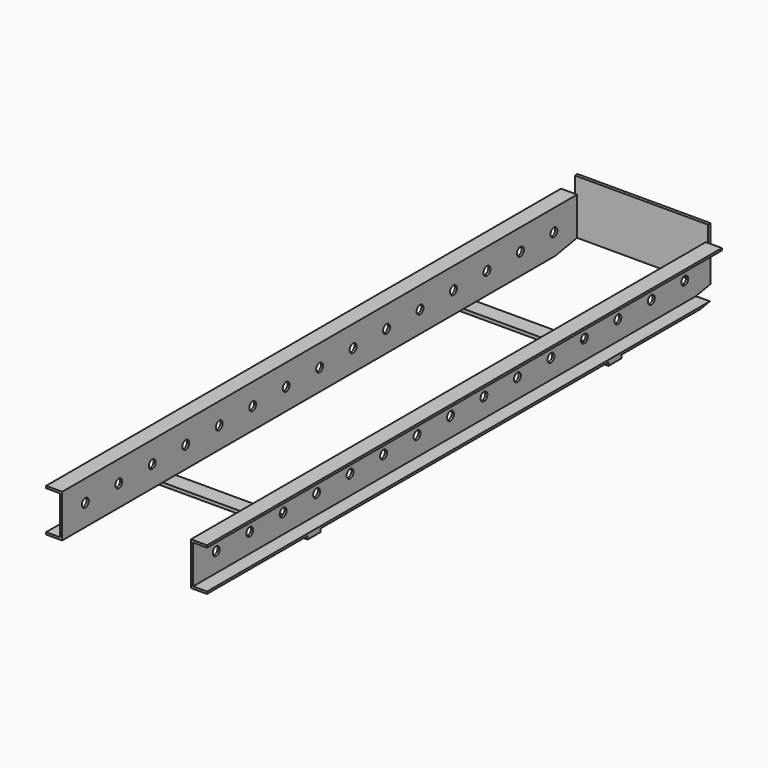
from build123d import *

# Parameters (mm, degrees)
F1_DEPTH    = 600
F2_R        = 4
F3_DEPTH    = 124
F5_W        = 150
F5_H        = 15
F6_DEPTH    = 3
F4_W        = 124
F4_H        = 55
F7_DEPTH    = 3
F8_T1_DEPTH = 271.3704583371


# Not quite as in the source:
# - a fillet or chamfer that OpenCascade refuses, or shapes differently, is made with other operations: its cross-section is extruded or revolved along the edge and cut away or added


with BuildPart() as f1:
    # F0 (on Front) → F1 (new body)
    with BuildSketch(Plane.XZ):
        Polygon((75, 17.5394031256), (75, 19.5394031256), (60, 19.5394031256), (60, -20.4605968744), (75, -20.4605968744), (75, -18.4605968744), (62, -18.4605968744), (62, 17.5394031256), align=None)
    extrude(amount=F1_DEPTH)


with BuildPart() as f1b:
    # F0 (on Front) → F1, piece 2 (new body)
    with BuildSketch(Plane.XZ):
        Polygon((-62, -18.4605968744), (-75, -18.4605968744), (-75, -20.4605968744), (-60, -20.4605968744), (-60, 19.5394031256), (-75, 19.5394031256), (-75, 17.5394031256), (-62, 17.5394031256), align=None)
    extrude(amount=F1_DEPTH)


with BuildPart() as f3_tool:
    # F2 (on face) → F3 (new body, through all)
    with BuildSketch(Plane.YZ.offset(62)):
        with Locations((-573.0000079556, -0.4398700211)):
            Circle(F2_R)
        with Locations((-534.0000079556, -0.4398700211)):
            Circle(F2_R)
        with Locations((-495.0000079556, -0.4398700211)):
            Circle(F2_R)
        with Locations((-456.0000079556, -0.4398700211)):
            Circle(F2_R)
        with Locations((-417.0000079556, -0.4398700211)):
            Circle(F2_R)
        with Locations((-378.0000079556, -0.4398700211)):
            Circle(F2_R)
        with Locations((-339.0000079556, -0.4398700211)):
            Circle(F2_R)
        with Locations((-300.0000079556, -0.4398700211)):
            Circle(F2_R)
        with Locations((-261.0000079556, -0.4398700211)):
            Circle(F2_R)
        with Locations((-222.0000079556, -0.4398700211)):
            Circle(F2_R)
        with Locations((-183.0000079556, -0.4398700211)):
            Circle(F2_R)
        with Locations((-144.0000079556, -0.4398700211)):
            Circle(F2_R)
        with Locations((-105.0000079556, -0.4398700211)):
            Circle(F2_R)
        with Locations((-66.0000079556, -0.4398700211)):
            Circle(F2_R)
        with Locations((-27.0000079556, -0.4398700211)):
            Circle(F2_R)
    extrude(amount=-F3_DEPTH)


with BuildPart() as f1_1:
    add(f1.part)

    # F3: cut by f3_tool
    add(f3_tool.part, mode=Mode.SUBTRACT)



with BuildPart() as f1b_1:
    add(f1b.part)

    # F3: cut by f3_tool
    add(f3_tool.part, mode=Mode.SUBTRACT)


with BuildPart() as f1_2:
    add(f1_1.part)

    add(f1b_1.part)  # F6 merges F1b
    # F5 (on face) → F6 (join)
    with BuildSketch(Plane(origin=(0, 0, -20.4605968744), x_dir=(1, 0, 0), z_dir=(0, 0, -1))):
        with Locations((0, 475.2312374115)):
            Rectangle(F5_W, F5_H)
        with Locations((0, 124.7687625885)):
            Rectangle(F5_W, F5_H)
    extrude(amount=F6_DEPTH)

    # F4 (on face) → F7 (join)
    with BuildSketch(Plane(origin=(0, 0, 0), x_dir=(-1, 0, 0), z_dir=(0, 1, 0))):
        with Locations((0, 7.0394031256)):
            Rectangle(F4_W, F4_H)
    extrude(amount=F7_DEPTH)

    # F8: chamfer of 5 x 28.3564090981 on 1 edges, made by hand

    # F8_s2 → F8_t1 (cut)
    with BuildSketch(Plane.YZ.offset(-135.6852291686)):
        Polygon((-25.3564090981, -20.4605968744), (3, -15.4605968744), (3, -20.4605968744), align=None)
    extrude(amount=F8_T1_DEPTH, mode=Mode.SUBTRACT)


solid = f1_2.part
